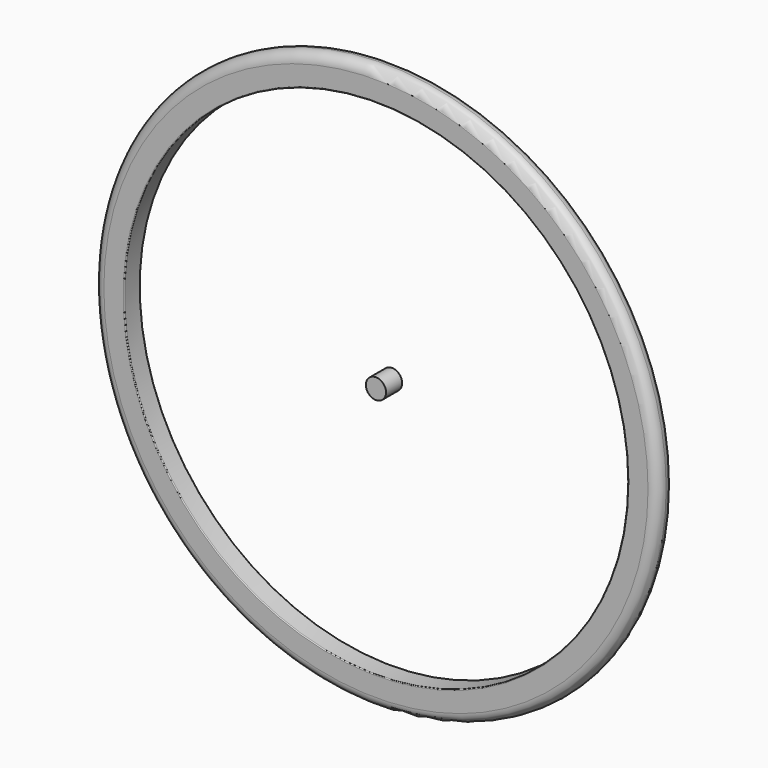
from build123d import *

# Parameters (mm, degrees)
F0_R     = 177.8
F1_DEPTH = 12.7
F2_R     = 158.75
F2_R_2   = 6.35
F3_DEPTH = 12.701
F4_R     = 6.34999
F5_R     = 0.508


# Not quite as in the source:
# - a fillet or chamfer is up to 0.001 mm smaller than in the source, because OpenCascade refuses the exact size


with BuildPart() as f1:
    # F0 (on Front) → F1 (new body)
    with BuildSketch(Plane.XZ):
        Circle(F0_R)
    extrude(amount=F1_DEPTH)

    # F2 (on face) → F3 (cut, through all)
    with BuildSketch(Plane.XZ.offset(12.7)):
        Circle(F2_R)
        Circle(F2_R_2, mode=Mode.SUBTRACT)
    extrude(amount=-F3_DEPTH, mode=Mode.SUBTRACT)

    # F4 (radius 6.35 in the source; OpenCascade refuses exactly that, so slightly less here)
    f4_edges = [f1.edges().sort_by_distance(p)[0] for p in [
        (-177.8, -12.7, 0),
        (-177.8, 0, 0),
    ]]
    fillet(f4_edges, radius=F4_R)

    # F5
    f5_edges = [f1.edges().sort_by_distance(p)[0] for p in [
        (-158.75, 0, 0),
        (-158.75, -12.7, 0),
    ]]
    fillet(f5_edges, radius=F5_R)


solid = f1.part
